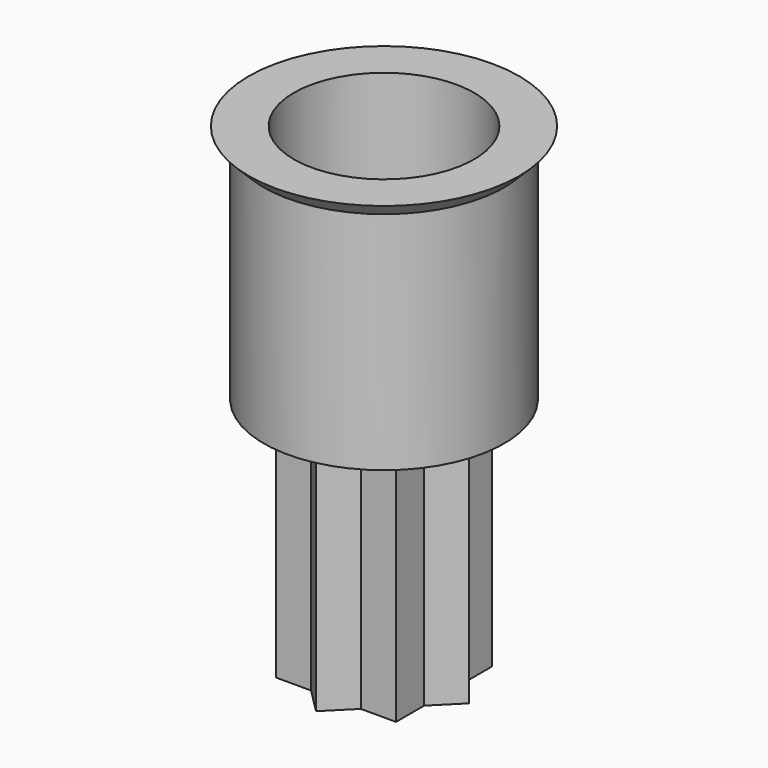
from build123d import *

# Parameters (mm, degrees)
F1_DEPTH      = 12.7
F4_DEPTH      = 25.4
F5_T1_DEPTH   = 2.0186367444
F5_T3_DEPTH   = 2.0186367444
F5_T5_DEPTH   = 2.0186367444
F5_T7_DEPTH   = 2.0186367444
F5_T9_DEPTH   = 2.0186367444
F5_T11_DEPTH  = 2.0186367444
F5_T13_DEPTH  = 2.0186367444
F5_T15_DEPTH  = 2.0186367444
F5_T17_DEPTH  = 2.0186367444
F5_T19_DEPTH  = 2.0186367444
F5_T21_DEPTH  = 2.0186367444
F5_T23_DEPTH  = 2.0186367444
F5_T29_DEPTH  = 2.214598988
F5_T35_DEPTH  = 2.214598988
F5_T44_DEPTH  = 2.214598988
F5_T50_DEPTH  = 2.214598988
F5_T59_DEPTH  = 2.214598988
F5_T65_DEPTH  = 2.214598988
F5_T74_DEPTH  = 2.214598988
F5_T80_DEPTH  = 2.214598988
F5_T89_DEPTH  = 2.214598988
F5_T95_DEPTH  = 2.214598988
F5_T104_DEPTH = 2.214598988
F5_T110_DEPTH = 2.214598988
F5_T119_DEPTH = 2.214598988
F5_T125_DEPTH = 2.214598988
F5_T134_DEPTH = 2.214598988
F5_T140_DEPTH = 2.214598988


# Not quite as in the source:
# - a fillet or chamfer that OpenCascade refuses, or shapes differently, is made with other operations: its cross-section is extruded or revolved along the edge and cut away or added


with BuildPart() as f1:
    # F0 (on Top) → F1 (new body)
    with BuildSketch(Plane.XY):
        Polygon((1.3151280605, -3.175), (3.175, -3.175), (3.175, -1.3151280605), (4.4901280605, 0), (3.175, 1.3151280605), (3.175, 3.175), (1.3151280605, 3.175), (0, 4.4901280605), (-1.3151280605, 3.175), (-3.175, 3.175), (-3.175, 1.3151280605), (-4.4901280605, 0), (-3.175, -1.3151280605), (-3.175, -3.175), (-1.3151280605, -3.175), (0, -4.4901280605), align=None)
        Polygon((3.1115, -1.2888254993), (3.1115, -3.1115), (1.2888254993, -3.1115), (0, -4.4003254993), (-1.2888254993, -3.1115), (-3.1115, -3.1115), (-3.1115, -1.2888254993), (-4.4003254993, 0), (-3.1115, 1.2888254993), (-3.1115, 3.1115), (-1.2888254993, 3.1115), (0, 4.4003254993), (1.2888254993, 3.1115), (3.1115, 3.1115), (3.1115, 1.2888254993), (4.4003254993, 0), align=None, mode=Mode.SUBTRACT)
    extrude(amount=-F1_DEPTH)

    # F2 (on Front) → F3 (revolve)
    with BuildSketch(Plane.XZ):
        Polygon((-6.35, 0), (0, 0), (0, 0.396875), (-4.7625, 0.396875), (-4.7625, 12.7), (-6.35, 12.7), (-6.35, 11.90625), align=None)
        Polygon((-7.14375, 12.7), (-6.35, 11.90625), (-6.35, 12.7), align=None)
    revolve(axis=Axis((0, 0, 0.1984375), (0, 0, 1)))

    # F4 (cut): a face of the model
    f4_faces = [f1.faces().sort_by_distance(p)[0] for p in [
        (0, 0, 0),
    ]]
    extrude(f4_faces, amount=-F4_DEPTH, mode=Mode.SUBTRACT)

    # F5: chamfer of 0.0762 on 16 edges, made by hand

    # F5_s2 → F5_t1 (cut)
    with BuildSketch(Plane(origin=(-0.772771019, -0.772771019, 0), x_dir=(0, 0, 1), z_dir=(-0.7071067812, -0.7071067812, 0))):
        Polygon((-12.7, -3.1877), (-12.6238, -3.1115), (-12.7, -3.1115), align=None)
    extrude(amount=F5_T1_DEPTH, mode=Mode.SUBTRACT)

    # F5_s4 → F5_t3 (cut)
    with BuildSketch(Plane.YZ.offset(1.0928632556)):
        Polygon((-3.1877, -12.7), (-3.1115, -12.6238), (-3.1115, -12.7), align=None)
        Polygon((3.1877, -12.7), (3.1115, -12.6238), (3.1115, -12.7), align=None)
    extrude(amount=F5_T3_DEPTH, mode=Mode.SUBTRACT)

    # F5_s6 → F5_t5 (cut)
    with BuildSketch(Plane.XZ.offset(1.0928632556)):
        Polygon((3.1877, -12.7), (3.1115, -12.6238), (3.1115, -12.7), align=None)
        Polygon((-3.1877, -12.7), (-3.1115, -12.6238), (-3.1115, -12.7), align=None)
    extrude(amount=F5_T5_DEPTH, mode=Mode.SUBTRACT)

    # F5_s8 → F5_t7 (cut)
    with BuildSketch(Plane(origin=(2.2001627497, 2.2001627497, 0), x_dir=(0, 0, 1), z_dir=(-0.7071067812, -0.7071067812, 0))):
        Polygon((-12.7, -3.1877), (-12.6238, -3.1115), (-12.7, -3.1115), align=None)
    extrude(amount=F5_T7_DEPTH, mode=Mode.SUBTRACT)

    # F5_s10 → F5_t9 (cut)
    with BuildSketch(Plane(origin=(0.772771019, -0.772771019, 0), x_dir=(0, 0, 1), z_dir=(0.7071067812, -0.7071067812, 0))):
        Polygon((-12.7, -3.1877), (-12.6238, -3.1115), (-12.7, -3.1115), align=None)
    extrude(amount=F5_T9_DEPTH, mode=Mode.SUBTRACT)

    # F5_s12 → F5_t11 (cut)
    with BuildSketch(Plane.XZ.offset(-3.1115)):
        Polygon((3.1877, -12.7), (3.1115, -12.6238), (3.1115, -12.7), align=None)
        Polygon((-3.1877, -12.7), (-3.1115, -12.6238), (-3.1115, -12.7), align=None)
    extrude(amount=F5_T11_DEPTH, mode=Mode.SUBTRACT)

    # F5_s14 → F5_t13 (cut)
    with BuildSketch(Plane(origin=(-2.2001627497, 2.2001627497, 0), x_dir=(0, 0, 1), z_dir=(0.7071067812, -0.7071067812, 0))):
        Polygon((-12.7, -3.1877), (-12.6238, -3.1115), (-12.7, -3.1115), align=None)
    extrude(amount=F5_T13_DEPTH, mode=Mode.SUBTRACT)

    # F5_s16 → F5_t15 (cut)
    with BuildSketch(Plane(origin=(0.772771019, 0.772771019, 0), x_dir=(0, 0, 1), z_dir=(0.7071067812, 0.7071067812, 0))):
        Polygon((-12.7, -3.1877), (-12.6238, -3.1115), (-12.7, -3.1115), align=None)
    extrude(amount=F5_T15_DEPTH, mode=Mode.SUBTRACT)

    # F5_s18 → F5_t17 (cut)
    with BuildSketch(Plane.YZ.offset(-3.1115)):
        Polygon((3.1877, -12.7), (3.1115, -12.6238), (3.1115, -12.7), align=None)
        Polygon((-3.1877, -12.7), (-3.1115, -12.6238), (-3.1115, -12.7), align=None)
    extrude(amount=F5_T17_DEPTH, mode=Mode.SUBTRACT)

    # F5_s20 → F5_t19 (cut)
    with BuildSketch(Plane(origin=(-2.2001627497, -2.2001627497, 0), x_dir=(0, 0, 1), z_dir=(0.7071067812, 0.7071067812, 0))):
        Polygon((-12.7, -3.1877), (-12.6238, -3.1115), (-12.7, -3.1115), align=None)
    extrude(amount=F5_T19_DEPTH, mode=Mode.SUBTRACT)

    # F5_s22 → F5_t21 (cut)
    with BuildSketch(Plane(origin=(-0.772771019, 0.772771019, 0), x_dir=(0, 0, 1), z_dir=(-0.7071067812, 0.7071067812, 0))):
        Polygon((-12.7, -3.1877), (-12.6238, -3.1115), (-12.7, -3.1115), align=None)
    extrude(amount=F5_T21_DEPTH, mode=Mode.SUBTRACT)

    # F5_s24 → F5_t23 (cut)
    with BuildSketch(Plane(origin=(2.2001627497, -2.2001627497, 0), x_dir=(0, 0, 1), z_dir=(-0.7071067812, 0.7071067812, 0))):
        Polygon((-12.7, -3.1877), (-12.6238, -3.1115), (-12.7, -3.1115), align=None)
    extrude(amount=F5_T23_DEPTH, mode=Mode.SUBTRACT)


with BuildPart() as f5_tool27:
    # F5_s28 → F5_t29 (new body)
    with BuildSketch(Plane(origin=(-0.772771019, -0.772771019, 0), x_dir=(0, 0, 1), z_dir=(-0.7071067812, -0.7071067812, 0))):
        Polygon((-12.7, -3.1877), (-12.6238, -3.1115), (-12.7, -3.1115), align=None)
    extrude(amount=F5_T29_DEPTH)

    split(bisect_by=Plane(origin=(2.2450640303, -2.2450640303, 0), x_dir=(0, 0, 1), z_dir=(-0.7071067812, 0.7071067812, 0)), keep=Keep.TOP)

    split(bisect_by=Plane(origin=(-2.2001627497, -2.2001627497, 0), x_dir=(0, 0, 1), z_dir=(-0.7071067812, -0.7071067812, 0)), keep=Keep.TOP)

    split(bisect_by=Plane(origin=(-2.2450640303, -2.2450640303, 0), x_dir=(0, 0, 1), z_dir=(0.7071067812, 0.7071067812, 0)), keep=Keep.TOP)


with BuildPart() as f5_tool33:
    # F5_s34 → F5_t35 (new body)
    with BuildSketch(Plane(origin=(2.338728981, -2.338728981, 0), x_dir=(0, 0, 1), z_dir=(-0.7071067812, 0.7071067812, 0))):
        Polygon((-12.7, -3.1877), (-12.6238, -3.1115), (-12.7, -3.1115), align=None)
    extrude(amount=F5_T35_DEPTH)

    split(bisect_by=Plane(origin=(2.2450640303, -2.2450640303, 0), x_dir=(0, 0, 1), z_dir=(-0.7071067812, 0.7071067812, 0)), keep=Keep.TOP)

    split(bisect_by=Plane(origin=(2.2001627497, -2.2001627497, 0), x_dir=(0, 0, 1), z_dir=(0.7071067812, -0.7071067812, 0)), keep=Keep.TOP)

    split(bisect_by=Plane(origin=(-2.2450640303, -2.2450640303, 0), x_dir=(0, 0, 1), z_dir=(0.7071067812, 0.7071067812, 0)), keep=Keep.TOP)


with BuildPart() as f5_tool27_1:
    add(f5_tool27.part)

    # F5_t39: intersect F5_tool33
    add(f5_tool33.part, mode=Mode.INTERSECT)


with BuildPart() as f1_1:
    add(f1.part)

    # F5_t25: cut F5_tool27
    add(f5_tool27_1.part, mode=Mode.SUBTRACT)


with BuildPart() as f5_tool42:
    # F5_s43 → F5_t44 (new body)
    with BuildSketch(Plane.XZ.offset(1.0928632556)):
        Polygon((3.1877, -12.7), (3.1115, -12.6238), (3.1115, -12.7), align=None)
    extrude(amount=F5_T44_DEPTH)

    split(bisect_by=Plane.XZ.offset(3.1115), keep=Keep.TOP)

    split(bisect_by=Plane.YZ.offset(3.175), keep=Keep.BOTTOM)

    split(bisect_by=Plane.XZ.offset(3.175), keep=Keep.BOTTOM)


with BuildPart() as f5_tool48:
    # F5_s49 → F5_t50 (new body)
    with BuildSketch(Plane.YZ.offset(3.3074622437)):
        Polygon((-3.1877, -12.7), (-3.1115, -12.6238), (-3.1115, -12.7), align=None)
    extrude(amount=-F5_T50_DEPTH)

    split(bisect_by=Plane.YZ.offset(3.1115), keep=Keep.TOP)

    split(bisect_by=Plane.YZ.offset(3.175), keep=Keep.BOTTOM)

    split(bisect_by=Plane.XZ.offset(3.175), keep=Keep.BOTTOM)


with BuildPart() as f5_tool42_1:
    add(f5_tool42.part)

    # F5_t54: intersect F5_tool48
    add(f5_tool48.part, mode=Mode.INTERSECT)


with BuildPart() as f1_2:
    add(f1_1.part)

    # F5_t40: cut F5_tool42
    add(f5_tool42_1.part, mode=Mode.SUBTRACT)


with BuildPart() as f5_tool57:
    # F5_s58 → F5_t59 (new body)
    with BuildSketch(Plane(origin=(0.772771019, -0.772771019, 0), x_dir=(0, 0, 1), z_dir=(0.7071067812, -0.7071067812, 0))):
        Polygon((-12.7, -3.1877), (-12.6238, -3.1115), (-12.7, -3.1115), align=None)
    extrude(amount=F5_T59_DEPTH)

    split(bisect_by=Plane(origin=(2.2001627497, -2.2001627497, 0), x_dir=(0, 0, 1), z_dir=(0.7071067812, -0.7071067812, 0)), keep=Keep.TOP)

    split(bisect_by=Plane(origin=(2.2450640303, 2.2450640303, 0), x_dir=(0, 0, 1), z_dir=(-0.7071067812, -0.7071067812, 0)), keep=Keep.TOP)

    split(bisect_by=Plane(origin=(2.2450640303, -2.2450640303, 0), x_dir=(0, 0, 1), z_dir=(-0.7071067812, 0.7071067812, 0)), keep=Keep.TOP)


with BuildPart() as f5_tool63:
    # F5_s64 → F5_t65 (new body)
    with BuildSketch(Plane(origin=(2.338728981, 2.338728981, 0), x_dir=(0, 0, 1), z_dir=(-0.7071067812, -0.7071067812, 0))):
        Polygon((-12.7, -3.1877), (-12.6238, -3.1115), (-12.7, -3.1115), align=None)
    extrude(amount=F5_T65_DEPTH)

    split(bisect_by=Plane(origin=(2.2001627497, 2.2001627497, 0), x_dir=(0, 0, 1), z_dir=(0.7071067812, 0.7071067812, 0)), keep=Keep.TOP)

    split(bisect_by=Plane(origin=(2.2450640303, 2.2450640303, 0), x_dir=(0, 0, 1), z_dir=(-0.7071067812, -0.7071067812, 0)), keep=Keep.TOP)

    split(bisect_by=Plane(origin=(2.2450640303, -2.2450640303, 0), x_dir=(0, 0, 1), z_dir=(-0.7071067812, 0.7071067812, 0)), keep=Keep.TOP)


with BuildPart() as f5_tool57_1:
    add(f5_tool57.part)

    # F5_t69: intersect F5_tool63
    add(f5_tool63.part, mode=Mode.INTERSECT)


with BuildPart() as f1_3:
    add(f1_2.part)

    # F5_t55: cut F5_tool57
    add(f5_tool57_1.part, mode=Mode.SUBTRACT)


with BuildPart() as f5_tool72:
    # F5_s73 → F5_t74 (new body)
    with BuildSketch(Plane.YZ.offset(1.0928632556)):
        Polygon((3.1877, -12.7), (3.1115, -12.6238), (3.1115, -12.7), align=None)
    extrude(amount=F5_T74_DEPTH)

    split(bisect_by=Plane.YZ.offset(3.1115), keep=Keep.TOP)

    split(bisect_by=Plane.XZ.offset(-3.175), keep=Keep.TOP)

    split(bisect_by=Plane.YZ.offset(3.175), keep=Keep.BOTTOM)


with BuildPart() as f5_tool78:
    # F5_s79 → F5_t80 (new body)
    with BuildSketch(Plane.XZ.offset(-3.3074622437)):
        Polygon((3.1877, -12.7), (3.1115, -12.6238), (3.1115, -12.7), align=None)
    extrude(amount=F5_T80_DEPTH)

    split(bisect_by=Plane.XZ.offset(-3.1115), keep=Keep.BOTTOM)

    split(bisect_by=Plane.XZ.offset(-3.175), keep=Keep.TOP)

    split(bisect_by=Plane.YZ.offset(3.175), keep=Keep.BOTTOM)


with BuildPart() as f5_tool72_1:
    add(f5_tool72.part)

    # F5_t84: intersect F5_tool78
    add(f5_tool78.part, mode=Mode.INTERSECT)


with BuildPart() as f1_4:
    add(f1_3.part)

    # F5_t70: cut F5_tool72
    add(f5_tool72_1.part, mode=Mode.SUBTRACT)


with BuildPart() as f5_tool87:
    # F5_s88 → F5_t89 (new body)
    with BuildSketch(Plane(origin=(-2.338728981, 2.338728981, 0), x_dir=(0, 0, 1), z_dir=(0.7071067812, -0.7071067812, 0))):
        Polygon((-12.7, -3.1877), (-12.6238, -3.1115), (-12.7, -3.1115), align=None)
    extrude(amount=F5_T89_DEPTH)

    split(bisect_by=Plane(origin=(-2.2001627497, 2.2001627497, 0), x_dir=(0, 0, 1), z_dir=(-0.7071067812, 0.7071067812, 0)), keep=Keep.TOP)

    split(bisect_by=Plane(origin=(-2.2450640303, 2.2450640303, 0), x_dir=(0, 0, 1), z_dir=(0.7071067812, -0.7071067812, 0)), keep=Keep.TOP)

    split(bisect_by=Plane(origin=(2.2450640303, 2.2450640303, 0), x_dir=(0, 0, 1), z_dir=(-0.7071067812, -0.7071067812, 0)), keep=Keep.TOP)


with BuildPart() as f5_tool93:
    # F5_s94 → F5_t95 (new body)
    with BuildSketch(Plane(origin=(0.772771019, 0.772771019, 0), x_dir=(0, 0, 1), z_dir=(0.7071067812, 0.7071067812, 0))):
        Polygon((-12.7, -3.1877), (-12.6238, -3.1115), (-12.7, -3.1115), align=None)
    extrude(amount=F5_T95_DEPTH)

    split(bisect_by=Plane(origin=(2.2001627497, 2.2001627497, 0), x_dir=(0, 0, 1), z_dir=(0.7071067812, 0.7071067812, 0)), keep=Keep.TOP)

    split(bisect_by=Plane(origin=(-2.2450640303, 2.2450640303, 0), x_dir=(0, 0, 1), z_dir=(0.7071067812, -0.7071067812, 0)), keep=Keep.TOP)

    split(bisect_by=Plane(origin=(2.2450640303, 2.2450640303, 0), x_dir=(0, 0, 1), z_dir=(-0.7071067812, -0.7071067812, 0)), keep=Keep.TOP)


with BuildPart() as f5_tool87_1:
    add(f5_tool87.part)

    # F5_t99: intersect F5_tool93
    add(f5_tool93.part, mode=Mode.INTERSECT)


with BuildPart() as f1_5:
    add(f1_4.part)

    # F5_t85: cut F5_tool87
    add(f5_tool87_1.part, mode=Mode.SUBTRACT)


with BuildPart() as f5_tool102:
    # F5_s103 → F5_t104 (new body)
    with BuildSketch(Plane.XZ.offset(-1.0928632556)):
        Polygon((-3.1877, -12.7), (-3.1115, -12.6238), (-3.1115, -12.7), align=None)
    extrude(amount=-F5_T104_DEPTH)

    split(bisect_by=Plane.XZ.offset(-3.1115), keep=Keep.BOTTOM)

    split(bisect_by=Plane.YZ.offset(-3.175), keep=Keep.TOP)

    split(bisect_by=Plane.XZ.offset(-3.175), keep=Keep.TOP)


with BuildPart() as f5_tool108:
    # F5_s109 → F5_t110 (new body)
    with BuildSketch(Plane.YZ.offset(-3.3074622437)):
        Polygon((3.1877, -12.7), (3.1115, -12.6238), (3.1115, -12.7), align=None)
    extrude(amount=F5_T110_DEPTH)

    split(bisect_by=Plane.YZ.offset(-3.1115), keep=Keep.BOTTOM)

    split(bisect_by=Plane.YZ.offset(-3.175), keep=Keep.TOP)

    split(bisect_by=Plane.XZ.offset(-3.175), keep=Keep.TOP)


with BuildPart() as f5_tool102_1:
    add(f5_tool102.part)

    # F5_t114: intersect F5_tool108
    add(f5_tool108.part, mode=Mode.INTERSECT)


with BuildPart() as f1_6:
    add(f1_5.part)

    # F5_t100: cut F5_tool102
    add(f5_tool102_1.part, mode=Mode.SUBTRACT)


with BuildPart() as f5_tool117:
    # F5_s118 → F5_t119 (new body)
    with BuildSketch(Plane(origin=(-0.772771019, 0.772771019, 0), x_dir=(0, 0, 1), z_dir=(-0.7071067812, 0.7071067812, 0))):
        Polygon((-12.7, -3.1877), (-12.6238, -3.1115), (-12.7, -3.1115), align=None)
    extrude(amount=F5_T119_DEPTH)

    split(bisect_by=Plane(origin=(-2.2001627497, 2.2001627497, 0), x_dir=(0, 0, 1), z_dir=(-0.7071067812, 0.7071067812, 0)), keep=Keep.TOP)

    split(bisect_by=Plane(origin=(-2.2450640303, -2.2450640303, 0), x_dir=(0, 0, 1), z_dir=(0.7071067812, 0.7071067812, 0)), keep=Keep.TOP)

    split(bisect_by=Plane(origin=(-2.2450640303, 2.2450640303, 0), x_dir=(0, 0, 1), z_dir=(0.7071067812, -0.7071067812, 0)), keep=Keep.TOP)


with BuildPart() as f5_tool123:
    # F5_s124 → F5_t125 (new body)
    with BuildSketch(Plane(origin=(-2.338728981, -2.338728981, 0), x_dir=(0, 0, 1), z_dir=(0.7071067812, 0.7071067812, 0))):
        Polygon((-12.7, -3.1877), (-12.6238, -3.1115), (-12.7, -3.1115), align=None)
    extrude(amount=F5_T125_DEPTH)

    split(bisect_by=Plane(origin=(-2.2001627497, -2.2001627497, 0), x_dir=(0, 0, 1), z_dir=(-0.7071067812, -0.7071067812, 0)), keep=Keep.TOP)

    split(bisect_by=Plane(origin=(-2.2450640303, -2.2450640303, 0), x_dir=(0, 0, 1), z_dir=(0.7071067812, 0.7071067812, 0)), keep=Keep.TOP)

    split(bisect_by=Plane(origin=(-2.2450640303, 2.2450640303, 0), x_dir=(0, 0, 1), z_dir=(0.7071067812, -0.7071067812, 0)), keep=Keep.TOP)


with BuildPart() as f5_tool117_1:
    add(f5_tool117.part)

    # F5_t129: intersect F5_tool123
    add(f5_tool123.part, mode=Mode.INTERSECT)


with BuildPart() as f1_7:
    add(f1_6.part)

    # F5_t115: cut F5_tool117
    add(f5_tool117_1.part, mode=Mode.SUBTRACT)


with BuildPart() as f5_tool132:
    # F5_s133 → F5_t134 (new body)
    with BuildSketch(Plane.YZ.offset(-1.0928632556)):
        Polygon((-3.1877, -12.7), (-3.1115, -12.6238), (-3.1115, -12.7), align=None)
    extrude(amount=-F5_T134_DEPTH)

    split(bisect_by=Plane.YZ.offset(-3.1115), keep=Keep.BOTTOM)

    split(bisect_by=Plane.XZ.offset(3.175), keep=Keep.BOTTOM)

    split(bisect_by=Plane.YZ.offset(-3.175), keep=Keep.TOP)


with BuildPart() as f5_tool138:
    # F5_s139 → F5_t140 (new body)
    with BuildSketch(Plane.XZ.offset(3.3074622437)):
        Polygon((-3.1877, -12.7), (-3.1115, -12.6238), (-3.1115, -12.7), align=None)
    extrude(amount=-F5_T140_DEPTH)

    split(bisect_by=Plane.XZ.offset(3.1115), keep=Keep.TOP)

    split(bisect_by=Plane.XZ.offset(3.175), keep=Keep.BOTTOM)

    split(bisect_by=Plane.YZ.offset(-3.175), keep=Keep.TOP)


with BuildPart() as f5_tool132_1:
    add(f5_tool132.part)

    # F5_t144: intersect F5_tool138
    add(f5_tool138.part, mode=Mode.INTERSECT)


with BuildPart() as f1_8:
    add(f1_7.part)

    # F5_t130: cut F5_tool132
    add(f5_tool132_1.part, mode=Mode.SUBTRACT)


solid = f1_8.part
